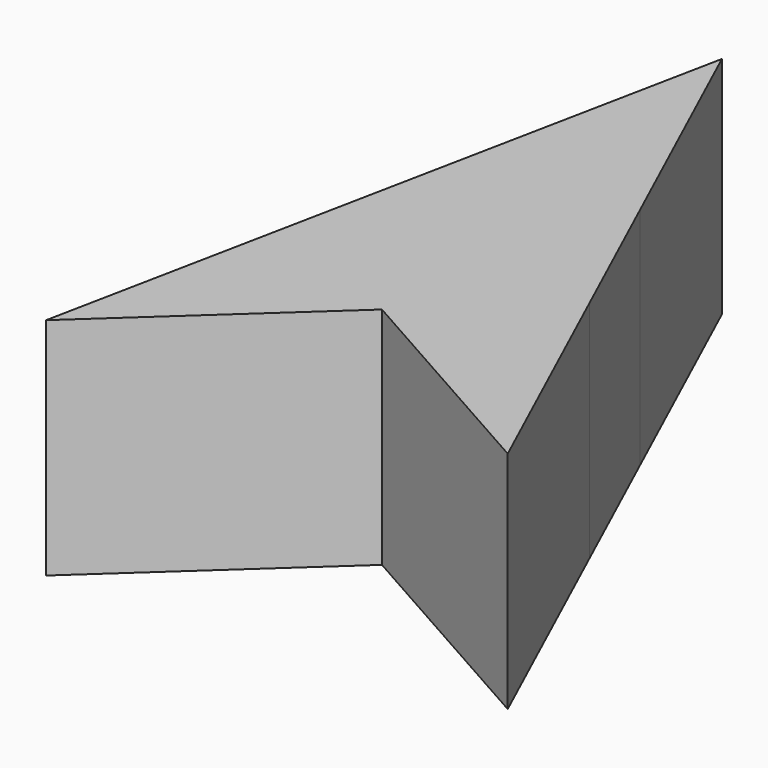
from build123d import *

# Parameters (mm, degrees)
F1_DEPTH = 25.4


with BuildPart() as f1:
    # F0 (on Top) → F1 (new body)
    with BuildSketch(Plane.XY):
        Polygon((-20.0724594905, -35.6141963687), (1.793154165, -15.5119398539), (-14.198616368, -6.4988439839), align=None)
        Polygon((1.793154165, -15.5119398539), (15.306846589, -3.0880620772), (7.6669972876, 13.6034125308), (-10.5683816736, 11.4954333843), (-14.198616368, -6.4988439839), align=None)
        Polygon((-10.5683816736, 11.4954333843), (7.6669972876, 13.6034125308), (-4.694538551, 40.6107857691), align=None)
        Polygon((27.6683824276, -30.0954353155), (15.306846589, -3.0880620772), (1.793154165, -15.5119398539), align=None)
    extrude(amount=F1_DEPTH)


solid = f1.part
